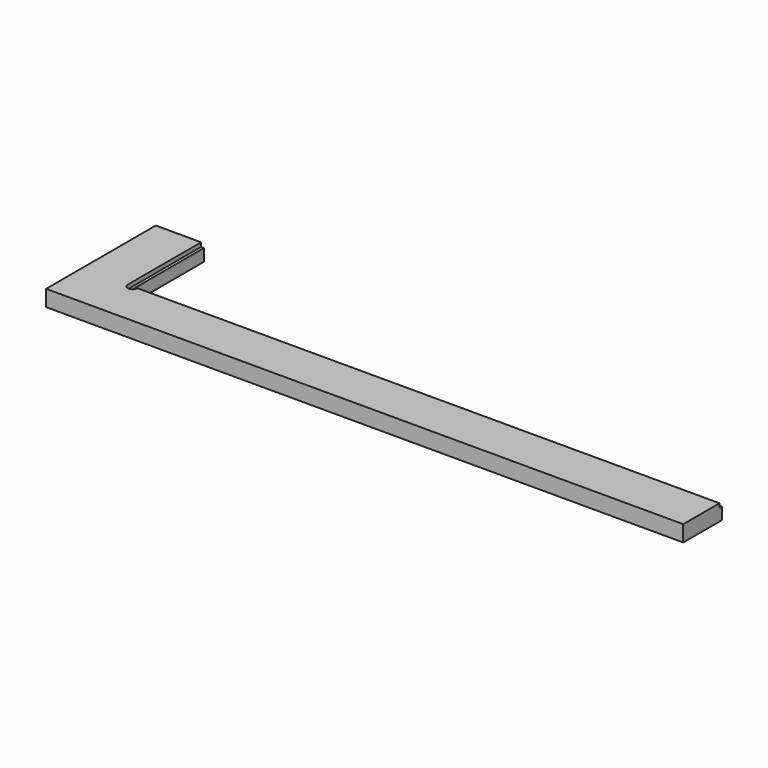
from build123d import *

# Parameters (mm, degrees)
F1_DEPTH = 19.05
F2_DEPTH = 6.35


# Not quite as in the source:
# - a length typed as a fraction of an inch, garbled in the dataset ("3 / 203.2 mm" for 3/8 in), is restored


with BuildPart() as f1:
    # F0 (on Top) → F1 (new body)
    with BuildSketch(Plane.XY):
        with BuildLine():
            Line((927.1, 0), (12.7, 0))
            ThreePointArc((12.7, 0), (12.1376302063, -2.6126302063), (10.5501302063, -4.7625))
            Line((10.5501302063, -4.7625), (927.1, -4.7625))
            Line((927.1, -4.7625), (927.1, 0))
        make_face()
        with BuildLine():
            Line((927.1, -4.7625), (10.5501302063, -4.7625))
            ThreePointArc((10.5501302063, -4.7625), (2.8938151032, -12.4188151032), (-4.7625, -4.7625))
            Line((-4.7625, -4.7625), (-4.7625, 139.7))
            Line((-4.7625, 139.7), (-76.2, 139.7))
            Line((-76.2, 139.7), (-76.2, -76.2))
            Line((-76.2, -76.2), (927.1, -76.2))
            Line((927.1, -76.2), (927.1, -4.7625))
        make_face()
        with BuildLine():
            ThreePointArc((-4.7625, -4.7625), (2.8938151032, -12.4188151032), (10.5501302063, -4.7625))
            ThreePointArc((10.5501302063, -4.7625), (3.7373697937, -5.7876302063), (0, 0))
            Line((0, 0), (0, 139.7))
            Line((0, 139.7), (-4.7625, 139.7))
            Line((-4.7625, 139.7), (-4.7625, -4.7625))
        make_face()
    extrude(amount=-F1_DEPTH)

    # F0 (on Top) → F2 (join)
    with BuildSketch(Plane.XY):
        with BuildLine():
            Line((927.1, -4.7625), (10.5501302063, -4.7625))
            ThreePointArc((10.5501302063, -4.7625), (2.8938151032, -12.4188151032), (-4.7625, -4.7625))
            Line((-4.7625, -4.7625), (-4.7625, 139.7))
            Line((-4.7625, 139.7), (-76.2, 139.7))
            Line((-76.2, 139.7), (-76.2, -76.2))
            Line((-76.2, -76.2), (927.1, -76.2))
            Line((927.1, -76.2), (927.1, -4.7625))
        make_face()
    extrude(amount=F2_DEPTH)


solid = f1.part
